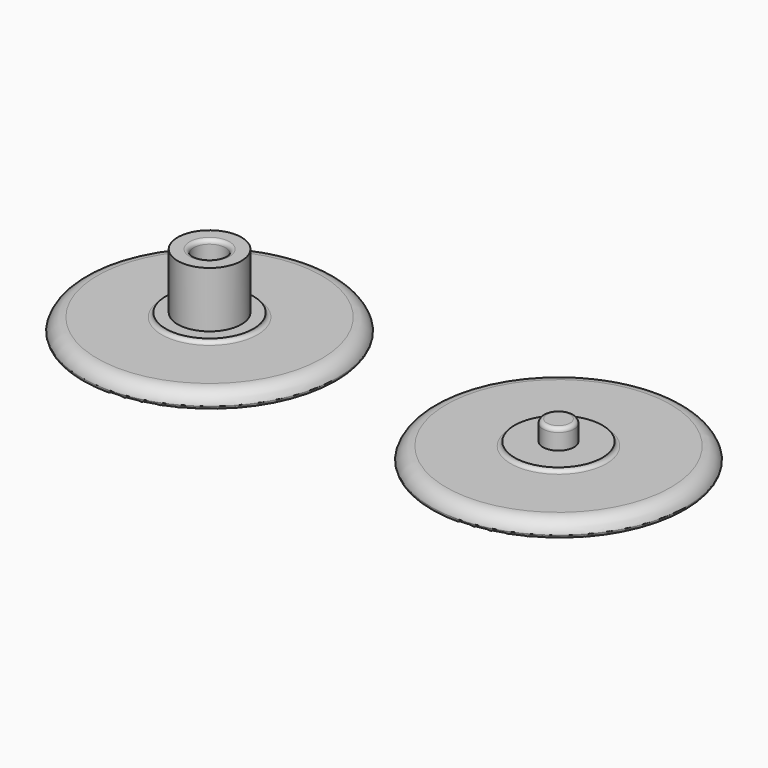
from build123d import *

# Parameters (mm, degrees)
F0_R     = 16
F0_R_2   = 5.5
F1_DEPTH = 2
F0_R_3   = 4
F2_DEPTH = 2.5
F0_R_4   = 1.95
F0_R_5   = 2
F3_DEPTH = 9.5
F4_DEPTH = 5
F5_R     = 0.49999
F5_2_R   = 0.49999


# Not quite as in the source:
# - a fillet or chamfer that OpenCascade refuses, or shapes differently, is made with other operations: its cross-section is extruded or revolved along the edge and cut away or added
# - a fillet or chamfer is up to 0.001 mm smaller than in the source, because OpenCascade refuses the exact size


with BuildPart() as f1:
    # F0 (on Top) → F1 (new body)
    with BuildSketch(Plane.XY):
        with Locations((-175.6076780854, 134.277998743)):
            Circle(F0_R)
        with Locations((-175.6076780854, 134.277998743)):
            Circle(F0_R_2, mode=Mode.SUBTRACT)
    extrude(amount=F1_DEPTH)

    # F0 (on Top) → F2 (join)
    with BuildSketch(Plane.XY):
        with Locations((-175.6076780854, 134.277998743)):
            Circle(F0_R_2)
        with Locations((-175.6076780854, 134.277998743)):
            Circle(F0_R_3, mode=Mode.SUBTRACT)
    extrude(amount=F2_DEPTH)



with BuildPart() as f1b:
    # F0 (on Top) → F1, piece 2 (new body)
    with BuildSketch(Plane.XY):
        with Locations((-131.8855119995, 134.277998743)):
            Circle(F0_R)
        with Locations((-131.8855119995, 134.277998743)):
            Circle(F0_R_2, mode=Mode.SUBTRACT)
    extrude(amount=F1_DEPTH)

    # F0 (on Top) → F2, piece 2 (join)
    with BuildSketch(Plane.XY):
        with Locations((-131.8855119995, 134.277998743)):
            Circle(F0_R_2)
        with Locations((-131.8855119995, 134.277998743)):
            Circle(F0_R_4, mode=Mode.SUBTRACT)
    extrude(amount=F2_DEPTH)

    # F0 (on Top) → F4 (join)
    with BuildSketch(Plane.XY):
        with Locations((-131.8855119995, 134.277998743)):
            Circle(F0_R_4)
    extrude(amount=F4_DEPTH)

    # F5#2 (radius 0.5 in the source; OpenCascade refuses exactly that, so slightly less here)
    f5_2_edges = [f1b.edges().sort_by_distance(p)[0] for p in [
        (-133.835512, 134.277999, 5),
        (-137.385512, 134.277999, 2),
        (-147.885512, 134.277999, 0),
    ]]
    fillet(f5_2_edges, radius=F5_2_R)

    # F6#2: fillet of radius 2 on 1 edges, made by hand

    # F6_2_s1 → F6_2_t2 (revolve, cut)
    with BuildSketch(Plane.XZ.offset(-134.277998743)):
        with BuildLine():
            ThreePointArc((-115.8855119995, 0.49999), (-116.5972573007, 1.5811356678), (-117.8220062546, 2))
            Line((-117.8220062546, 2), (-117.8220062546, 2.04))
            Line((-117.8220062546, 2.04), (-115.8855119995, 2.04))
            Line((-115.8855119995, 2.04), (-115.8455119995, 2))
            ThreePointArc((-115.8455119995, 2), (-115.8455119995, 1.249995), (-115.8467821144, 0.5099898))
            Line((-115.8467821144, 0.5099898), (-115.8855119995, 0.49999))
        make_face()
    revolve(axis=Axis((-131.8855119995, 134.277998743, 2), (0, 0, 1)), mode=Mode.SUBTRACT)


with BuildPart() as f2:
    # F0 (on Top) → F2, piece 3 (new body)
    with BuildSketch(Plane.XY):
        with Locations((-175.6076780854, 134.277998743)):
            Circle(F0_R_5)
    extrude(amount=F2_DEPTH)


with BuildPart() as f1_1:
    add(f1.part)

    add(f2.part)  # F3 merges F2
    # F0 (on Top) → F3 (join)
    with BuildSketch(Plane.XY):
        with Locations((-175.6076780854, 134.277998743)):
            Circle(F0_R_3)
        with Locations((-175.6076780854, 134.277998743)):
            Circle(F0_R_5, mode=Mode.SUBTRACT)
    extrude(amount=F3_DEPTH)

    # F5 (radius 0.5 in the source; OpenCascade refuses exactly that, so slightly less here)
    f5_edges = [f1_1.edges().sort_by_distance(p)[0] for p in [
        (-177.607678, 134.277999, 9.5),
        (-181.107678, 134.277999, 2),
        (-191.607678, 134.277999, 0),
    ]]
    fillet(f5_edges, radius=F5_R)

    # F6: fillet of radius 2 on 1 edges, made by hand

    # F6_s1 → F6_t2 (revolve, cut)
    with BuildSketch(Plane.XZ.offset(-134.277998743)):
        with BuildLine():
            ThreePointArc((-159.6076780854, 0.49999), (-160.3194233866, 1.5811356678), (-161.5441723405, 2))
            Line((-161.5441723405, 2), (-161.5441723405, 2.04))
            Line((-161.5441723405, 2.04), (-159.6076780854, 2.04))
            Line((-159.6076780854, 2.04), (-159.5676780854, 2))
            ThreePointArc((-159.5676780854, 2), (-159.5676780854, 1.249995), (-159.5689482003, 0.5099898))
            Line((-159.5689482003, 0.5099898), (-159.6076780854, 0.49999))
        make_face()
    revolve(axis=Axis((-175.6076780854, 134.277998743, 2), (0, 0, 1)), mode=Mode.SUBTRACT)


solid = Compound([f1b.part, f1_1.part])
